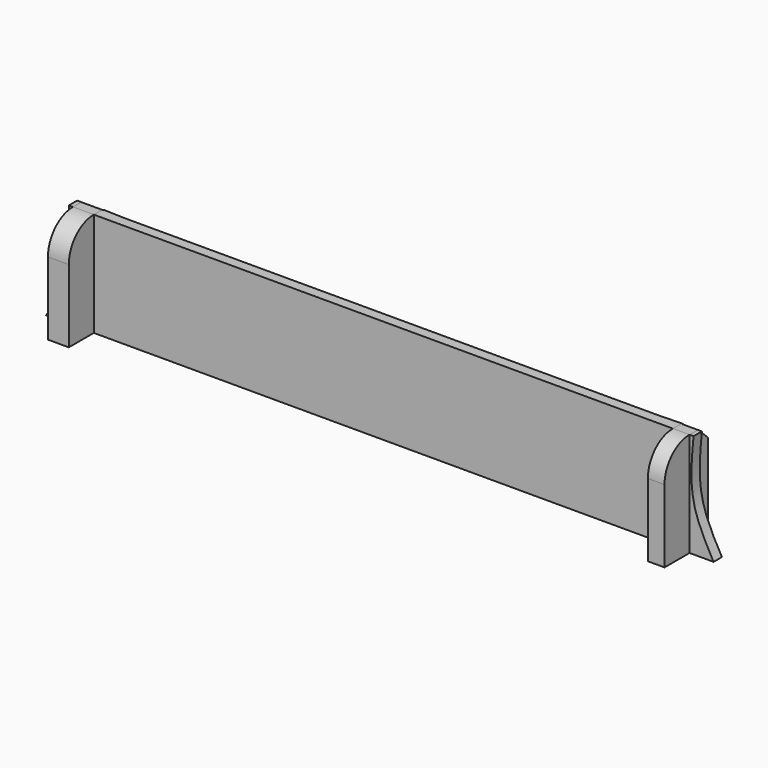
from build123d import *

# Parameters (mm, degrees)
F2_DEPTH  = 12.7
F3_DEPTH  = 375.92
F4_DEPTH  = 355.6
F5_DEPTH  = 751.84
F6_DEPTH  = 726.44
F8_DEPTH  = 127
F9_SIZE   = 13.97
F9_2_SIZE = 13.97
F10_R     = 38.1
F10_2_R   = 38.1


with BuildPart() as f2:
    # F0 (on Front) → F2 (new body)
    with BuildSketch(Plane.XZ):
        with BuildLine():
            Line((380.8272553887, 0), (0, 0))
            Line((0, 0), (-381, 0))
            add(Edge.make_bspline(
                [(-381, 0), (-378.5180144942, -24.1278339391), (-373.6845366605, -71.2463261626), (-397.2052409969, -108.7811267769), (-408.6969792843, -127)],
                knots=[0, 0, 0, 0, 0.5119270914, 1, 1, 1, 1], degree=3))
            Line((-408.6969792843, -127), (405.2553772926, -127))
            add(Edge.make_bspline(
                [(380.8272553887, 0), (378.6026539617, -24.075771659), (374.2937220743, -70.8487324495), (395.1306170121, -108.7180910096), (405.2553772926, -127)],
                knots=[0, 0, 0, 0, 0.5146236499, 1, 1, 1, 1], degree=3))
        make_face()
    extrude(amount=F2_DEPTH)


with BuildPart() as f3:
    # F1 (on Right) → F3 (new body)
    with BuildSketch(Plane.YZ):
        Polygon((15.24, -14.2560294469), (0, 0), (-50.8, 0), (-50.8, -75.6412135187), (-50.8, -127), (15.24, -127), (15.24, -75.6412135187), align=None)
    extrude(amount=F3_DEPTH)

    # F4 (cut): a face of the model
    f4_faces = [f3.faces().sort_by_distance(p)[0] for p in [
        (0, -18.1466325136, -64.2708991879),
    ]]
    extrude(f4_faces, amount=-F4_DEPTH, mode=Mode.SUBTRACT)


with BuildPart() as f5:
    # F5 (new): a face of the model
    f5_faces = [f3.part.faces().sort_by_distance(p)[0] for p in [
        (375.92, -18.1466325136, -64.2708991879),
    ]]
    extrude(f5_faces, amount=-F5_DEPTH)

    # F6 (cut): a face of the model
    f6_faces = [f3.part.faces().sort_by_distance(p)[0] for p in [
        (375.92, -18.1466325136, -64.2708991879),
    ]]
    extrude(f6_faces, amount=-F6_DEPTH, mode=Mode.SUBTRACT)

    # F10#2
    f10_2_edges = [f5.edges().sort_by_distance(p)[0] for p in [
        (-363.22, -50.8, 0),
    ]]
    fillet(f10_2_edges, radius=F10_2_R)


with BuildPart() as f8:
    # F7 (on Top) → F8 (new body)
    with BuildSketch(Plane.XY):
        Polygon((-349.5178818703, 0), (0, 0), (-349.5178818703, 15.0260068476), align=None)
    extrude(amount=-F8_DEPTH)

    # F9
    f9_edges = [f8.edges().sort_by_distance(p)[0] for p in [
        (-174.758941, 7.513003, 0),
    ]]
    chamfer(f9_edges, length=F9_SIZE)


with BuildPart() as f8b:
    # F7 (on Top) → F8, piece 2 (new body)
    with BuildSketch(Plane.XY):
        Polygon((356.3379347324, 15.0260068476), (0, 0), (356.3379347324, 0), align=None)
    extrude(amount=-F8_DEPTH)

    # F9#2
    f9_2_edges = [f8b.edges().sort_by_distance(p)[0] for p in [
        (178.168967, 7.513003, 0),
    ]]
    chamfer(f9_2_edges, length=F9_2_SIZE)


with BuildPart() as f3_1:
    add(f3.part)

    # F10
    f10_edges = [f3_1.edges().sort_by_distance(p)[0] for p in [
        (365.76, -50.8, 0),
    ]]
    fillet(f10_edges, radius=F10_R)


solid = Compound([f2.part, f5.part, f8.part, f8b.part, f3_1.part])
